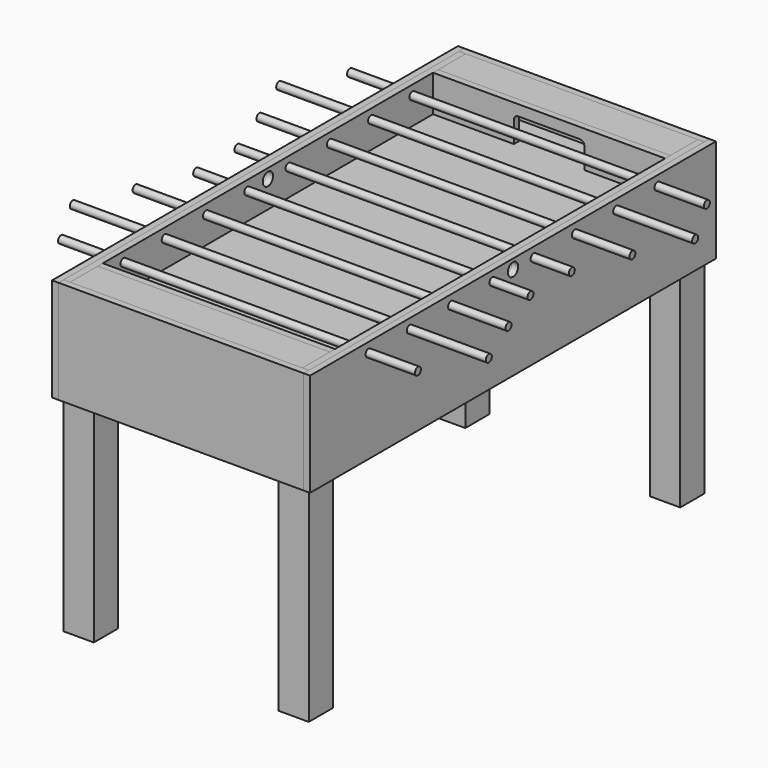
from build123d import *

# Parameters (mm, degrees)
F0_W      = 723.9
F0_H      = 1257.3
F1_DEPTH  = 19.05
F3_DEPTH  = 107.95
F4_DEPTH  = 107.95
F2_W      = 685.8
F2_H      = 19.05
F5_DEPTH  = 107.95
F6_DEPTH  = 107.95
F10_DEPTH = 1257.301
F11_DEPTH = 527.05
F8_R      = 11.1125
F12_DEPTH = 614.3625
F13_DEPTH = 550.8625
F14_DEPTH = 493.7125
F15_W     = 723.9
F15_H     = 1257.3
F15_H_2   = 101.6
F16_DEPTH = 19.05
F17_W     = 19.05
F17_H     = 101.6
F18_DEPTH = 107.95
F19_W     = 685.8
F19_H     = 19.05
F20_DEPTH = 88.9
F21_W     = 88.9
F21_H     = 88.9
F22_DEPTH = 787.4
F23_W     = 685.8
F23_H     = 101.6
F24_DEPTH = 19.05
F26_DEPTH = 304.8
F27_DEPTH = 304.8
F28_DEPTH = 420.624


with BuildPart() as f1:
    # F0 (on Top) → F1 (new body)
    with BuildSketch(Plane.XY):
        with Locations((297.7294597745, 583.4037639737)):
            Rectangle(F0_W, F0_H)
    extrude(amount=-F1_DEPTH)

    # F15 (on face) → F16 (join)
    with BuildSketch(Plane.XY):
        with Locations((297.7294597745, 583.4037639737)):
            Rectangle(F15_W, F15_H)
        with Locations((297.7294597745, -96.0462360263)):
            Rectangle(F15_W, F15_H_2)
        with Locations((297.7294597745, 1262.8537639737)):
            Rectangle(F15_W, F15_H_2)
    extrude(amount=-F16_DEPTH)


with BuildPart() as f3:
    # F2 (on face) → F3 (new body)
    with BuildSketch(Plane.XY):
        Polygon((640.6294597745, -26.1962360263), (640.6294597745, -45.2462360263), (659.6794597745, -45.2462360263), (659.6794597745, 1212.0537639737), (640.6294597745, 1212.0537639737), (640.6294597745, 1193.0037639737), align=None)
    extrude(amount=F3_DEPTH)

    # F17 (on face) → F18 (join, through all)
    with BuildSketch(Plane.XY):
        with Locations((650.1544597745, 1262.8537639737)):
            Rectangle(F17_W, F17_H)
        with Locations((650.1544597745, -96.0462360263)):
            Rectangle(F17_W, F17_H)
    extrude(amount=F18_DEPTH)


with BuildPart() as f4:
    # F2 (on face) → F4 (new body)
    with BuildSketch(Plane.XY):
        Polygon((-64.2205402255, 1212.0537639737), (-64.2205402255, -45.2462360263), (-45.1705402255, -45.2462360263), (-45.1705402255, -26.1962360263), (-45.1705402255, 1193.0037639737), (-45.1705402255, 1212.0537639737), align=None)
    extrude(amount=F4_DEPTH)

    # F17 (on face) → F18, piece 2 (join, through all)
    with BuildSketch(Plane.XY):
        with Locations((-54.6955402255, 1262.8537639737)):
            Rectangle(F17_W, F17_H)
        with Locations((-54.6955402255, -96.0462360263)):
            Rectangle(F17_W, F17_H)
    extrude(amount=F18_DEPTH)


with BuildPart() as f5:
    # F2 (on face) → F5 (new body)
    with BuildSketch(Plane.XY):
        with Locations((297.7294597745, -35.7212360263)):
            Rectangle(F2_W, F2_H)
    extrude(amount=F5_DEPTH)


with BuildPart() as f6:
    # F2 (on face) → F6 (new body)
    with BuildSketch(Plane.XY):
        with Locations((297.7294597745, 1202.5287639737)):
            Rectangle(F2_W, F2_H)
    extrude(amount=F6_DEPTH)


with BuildPart() as f10_tool:
    # F9 (on face) → F10 (new body, through all)
    with BuildSketch(Plane(origin=(0, 1212.0537639737, 0), x_dir=(-1, 0, 0), z_dir=(0, 1, 0))):
        with BuildLine():
            Line((-401.7107097745, 0), (-297.7294597745, 0))
            Line((-297.7294597745, 0), (-297.7294597745, 76.2))
            Line((-297.7294597745, 76.2), (-389.0107097745, 76.2))
            ThreePointArc((-389.0107097745, 76.2), (-397.9909658956, 72.4802561211), (-401.7107097745, 63.5))
            Line((-401.7107097745, 63.5), (-401.7107097745, 0))
        make_face()
        with BuildLine():
            Line((-297.7294597745, 76.2), (-297.7294597745, 0))
            Line((-297.7294597745, 0), (-193.7482097745, 0))
            Line((-193.7482097745, 0), (-193.7482097745, 63.5))
            ThreePointArc((-193.7482097745, 63.5), (-197.4679536534, 72.4802561211), (-206.4482097745, 76.2))
            Line((-206.4482097745, 76.2), (-297.7294597745, 76.2))
        make_face()
    extrude(amount=-F10_DEPTH)


with BuildPart() as f5_1:
    add(f5.part)

    # F10: cut by f10_tool
    add(f10_tool.part, mode=Mode.SUBTRACT)


with BuildPart() as f6_1:
    add(f6.part)

    # F10: cut by f10_tool
    add(f10_tool.part, mode=Mode.SUBTRACT)


with BuildPart() as f11:
    # F8 (on offset) → F11 (new body, symmetric)
    with BuildSketch(Plane.YZ.offset(297.7294597745)):
        with BuildLine():
            ThreePointArc((1127.9162639737, 79.375), (1116.8037639737, 90.4875), (1105.6912639737, 79.375))
            ThreePointArc((1105.6912639737, 79.375), (1116.8037639737, 68.2625), (1127.9162639737, 79.375))
        make_face()
    extrude(amount=F11_DEPTH, both=True)


with BuildPart() as f11b:
    # F8 (on offset) → F11, piece 2 (new body, symmetric)
    with BuildSketch(Plane.YZ.offset(297.7294597745)):
        with Locations((50.0037639737, 79.375)):
            Circle(F8_R)
    extrude(amount=F11_DEPTH, both=True)


with BuildPart() as f12:
    # F8 (on offset) → F12 (new body, symmetric)
    with BuildSketch(Plane.YZ.offset(297.7294597745)):
        with BuildLine():
            Line((964.4037639737, 79.375), (953.2912639737, 79.375))
            ThreePointArc((953.2912639737, 79.375), (964.4037639737, 68.2625), (975.5162639737, 79.375))
            Line((975.5162639737, 79.375), (964.4037639737, 79.375))
        make_face()
        with BuildLine():
            ThreePointArc((975.5162639737, 79.375), (964.4037639737, 90.4875), (953.2912639737, 79.375))
            Line((953.2912639737, 79.375), (964.4037639737, 79.375))
            Line((964.4037639737, 79.375), (975.5162639737, 79.375))
        make_face()
    extrude(amount=F12_DEPTH, both=True)


with BuildPart() as f12b:
    # F8 (on offset) → F12, piece 2 (new body, symmetric)
    with BuildSketch(Plane.YZ.offset(297.7294597745)):
        with BuildLine():
            ThreePointArc((191.2912639737, 79.375), (202.4037639737, 68.2625), (213.5162639737, 79.375))
            Line((213.5162639737, 79.375), (202.4037639737, 79.375))
            Line((202.4037639737, 79.375), (191.2912639737, 79.375))
        make_face()
        with BuildLine():
            Line((202.4037639737, 79.375), (213.5162639737, 79.375))
            ThreePointArc((213.5162639737, 79.375), (202.4037639737, 90.4875), (191.2912639737, 79.375))
            Line((191.2912639737, 79.375), (202.4037639737, 79.375))
        make_face()
    extrude(amount=F12_DEPTH, both=True)


with BuildPart() as f13:
    # F8 (on offset) → F13 (new body, symmetric)
    with BuildSketch(Plane.YZ.offset(297.7294597745)):
        with BuildLine():
            Line((812.0037639737, 79.375), (800.8912639737, 79.375))
            ThreePointArc((800.8912639737, 79.375), (812.0037639737, 68.2625), (823.1162639737, 79.375))
            Line((823.1162639737, 79.375), (812.0037639737, 79.375))
        make_face()
        with BuildLine():
            ThreePointArc((823.1162639737, 79.375), (812.0037639737, 90.4875), (800.8912639737, 79.375))
            Line((800.8912639737, 79.375), (812.0037639737, 79.375))
            Line((812.0037639737, 79.375), (823.1162639737, 79.375))
        make_face()
    extrude(amount=F13_DEPTH, both=True)


with BuildPart() as f13b:
    # F8 (on offset) → F13, piece 2 (new body, symmetric)
    with BuildSketch(Plane.YZ.offset(297.7294597745)):
        with BuildLine():
            Line((354.8037639737, 79.375), (365.9162639737, 79.375))
            ThreePointArc((365.9162639737, 79.375), (354.8037639737, 90.4875), (343.6912639737, 79.375))
            Line((343.6912639737, 79.375), (354.8037639737, 79.375))
        make_face()
        with BuildLine():
            ThreePointArc((343.6912639737, 79.375), (354.8037639737, 68.2625), (365.9162639737, 79.375))
            Line((365.9162639737, 79.375), (354.8037639737, 79.375))
            Line((354.8037639737, 79.375), (343.6912639737, 79.375))
        make_face()
    extrude(amount=F13_DEPTH, both=True)


with BuildPart() as f14:
    # F8 (on offset) → F14 (new body, symmetric)
    with BuildSketch(Plane.YZ.offset(297.7294597745)):
        with BuildLine():
            ThreePointArc((496.0912639737, 79.375), (507.2037639737, 68.2625), (518.3162639737, 79.375))
            Line((518.3162639737, 79.375), (507.2037639737, 79.375))
            Line((507.2037639737, 79.375), (496.0912639737, 79.375))
        make_face()
        with BuildLine():
            Line((507.2037639737, 79.375), (518.3162639737, 79.375))
            ThreePointArc((518.3162639737, 79.375), (507.2037639737, 90.4875), (496.0912639737, 79.375))
            Line((496.0912639737, 79.375), (507.2037639737, 79.375))
        make_face()
    extrude(amount=F14_DEPTH, both=True)


with BuildPart() as f14b:
    # F8 (on offset) → F14, piece 2 (new body, symmetric)
    with BuildSketch(Plane.YZ.offset(297.7294597745)):
        with BuildLine():
            Line((659.6037639737, 79.375), (648.4912639737, 79.375))
            ThreePointArc((648.4912639737, 79.375), (659.6037639737, 68.2625), (670.7162639737, 79.375))
            Line((670.7162639737, 79.375), (659.6037639737, 79.375))
        make_face()
        with BuildLine():
            ThreePointArc((670.7162639737, 79.375), (659.6037639737, 90.4875), (648.4912639737, 79.375))
            Line((648.4912639737, 79.375), (659.6037639737, 79.375))
            Line((659.6037639737, 79.375), (670.7162639737, 79.375))
        make_face()
    extrude(amount=F14_DEPTH, both=True)


with BuildPart() as f20:
    # F19 (on face) → F20 (new body)
    with BuildSketch(Plane.XY):
        with Locations((297.7294597745, -137.3212360263)):
            Rectangle(F19_W, F19_H)
    extrude(amount=F20_DEPTH)


with BuildPart() as f20b:
    # F19 (on face) → F20, piece 2 (new body)
    with BuildSketch(Plane.XY):
        with Locations((297.7294597745, 1304.1287639737)):
            Rectangle(F19_W, F19_H)
    extrude(amount=F20_DEPTH)


with BuildPart() as f22:
    # F21 (on face) → F22 (new body)
    with BuildSketch(Plane(origin=(0, 0, -19.05), x_dir=(1, 0, 0), z_dir=(0, 0, -1))):
        with Locations((-19.7705402255, -1269.2037639737)):
            Rectangle(F21_W, F21_H)
    extrude(amount=F22_DEPTH)


with BuildPart() as f22b:
    # F21 (on face) → F22, piece 2 (new body)
    with BuildSketch(Plane(origin=(0, 0, -19.05), x_dir=(1, 0, 0), z_dir=(0, 0, -1))):
        with Locations((-19.7705402255, 102.3962360263)):
            Rectangle(F21_W, F21_H)
    extrude(amount=F22_DEPTH)


with BuildPart() as f22c:
    # F21 (on face) → F22, piece 3 (new body)
    with BuildSketch(Plane(origin=(0, 0, -19.05), x_dir=(1, 0, 0), z_dir=(0, 0, -1))):
        with Locations((615.2294597745, -1269.2037639737)):
            Rectangle(F21_W, F21_H)
    extrude(amount=F22_DEPTH)


with BuildPart() as f22d:
    # F21 (on face) → F22, piece 4 (new body)
    with BuildSketch(Plane(origin=(0, 0, -19.05), x_dir=(1, 0, 0), z_dir=(0, 0, -1))):
        with Locations((615.2294597745, 102.3962360263)):
            Rectangle(F21_W, F21_H)
    extrude(amount=F22_DEPTH)


with BuildPart() as f24:
    # F23 (on face) → F24 (new body)
    with BuildSketch(Plane.XY.offset(88.9)):
        with Locations((297.7294597745, -96.0462360263)):
            Rectangle(F23_W, F23_H)
    extrude(amount=F24_DEPTH)


with BuildPart() as f24b:
    # F23 (on face) → F24, piece 2 (new body)
    with BuildSketch(Plane.XY.offset(88.9)):
        with Locations((297.7294597745, 1262.8537639737)):
            Rectangle(F23_W, F23_H)
    extrude(amount=F24_DEPTH)


with BuildPart() as f26:
    # F25 (on face) → F26 (new body)
    with BuildSketch(Plane.XY.offset(107.95)):
        Polygon((659.6794597745, -165.8962360263), (659.6794597745, -146.8462360263), (640.6294597745, -146.8462360263), (-45.1705402255, -146.8462360263), (-64.2205402255, -146.8462360263), (-64.2205402255, -165.8962360263), align=None)
    extrude(amount=-F26_DEPTH)


with BuildPart() as f26b:
    # F25 (on face) → F26, piece 2 (new body)
    with BuildSketch(Plane.XY.offset(107.95)):
        Polygon((640.6294597745, 1313.6537639737), (659.6794597745, 1313.6537639737), (659.6794597745, 1332.7037639737), (-64.2205402255, 1332.7037639737), (-64.2205402255, 1313.6537639737), (-45.1705402255, 1313.6537639737), align=None)
    extrude(amount=-F26_DEPTH)


with BuildPart() as f27:
    # F25 (on face) → F27 (new body)
    with BuildSketch(Plane.XY.offset(107.95)):
        Polygon((659.6794597745, 1313.6537639737), (659.6794597745, -146.8462360263), (659.6794597745, -165.8962360263), (678.7294597745, -165.8962360263), (678.7294597745, 1332.7037639737), (659.6794597745, 1332.7037639737), align=None)
    extrude(amount=-F27_DEPTH)


with BuildPart() as f27b:
    # F25 (on face) → F27, piece 2 (new body)
    with BuildSketch(Plane.XY.offset(107.95)):
        Polygon((-83.2705402255, -165.8962360263), (-64.2205402255, -165.8962360263), (-64.2205402255, -146.8462360263), (-64.2205402255, 1313.6537639737), (-64.2205402255, 1332.7037639737), (-83.2705402255, 1332.7037639737), align=None)
    extrude(amount=-F27_DEPTH)


with BuildPart() as f28_tool:
    # F8 (on offset) → F28 (new body, symmetric)
    with BuildSketch(Plane.YZ.offset(297.7294597745)):
        with BuildLine():
            ThreePointArc((564.3537639737, 79.375), (569.9333797921, 65.9046158184), (583.4037639737, 60.325))
            Line((583.4037639737, 60.325), (583.4037639737, 79.375))
            Line((583.4037639737, 79.375), (564.3537639737, 79.375))
        make_face()
        with Locations((50.0037639737, 79.375)):
            Circle(F8_R)
        with BuildLine():
            ThreePointArc((191.2912639737, 79.375), (202.4037639737, 68.2625), (213.5162639737, 79.375))
            Line((213.5162639737, 79.375), (202.4037639737, 79.375))
            Line((202.4037639737, 79.375), (191.2912639737, 79.375))
        make_face()
        with BuildLine():
            Line((202.4037639737, 79.375), (213.5162639737, 79.375))
            ThreePointArc((213.5162639737, 79.375), (202.4037639737, 90.4875), (191.2912639737, 79.375))
            Line((191.2912639737, 79.375), (202.4037639737, 79.375))
        make_face()
        with BuildLine():
            ThreePointArc((343.6912639737, 79.375), (354.8037639737, 68.2625), (365.9162639737, 79.375))
            Line((365.9162639737, 79.375), (354.8037639737, 79.375))
            Line((354.8037639737, 79.375), (343.6912639737, 79.375))
        make_face()
        with BuildLine():
            Line((354.8037639737, 79.375), (365.9162639737, 79.375))
            ThreePointArc((365.9162639737, 79.375), (354.8037639737, 90.4875), (343.6912639737, 79.375))
            Line((343.6912639737, 79.375), (354.8037639737, 79.375))
        make_face()
        with BuildLine():
            ThreePointArc((496.0912639737, 79.375), (507.2037639737, 68.2625), (518.3162639737, 79.375))
            Line((518.3162639737, 79.375), (507.2037639737, 79.375))
            Line((507.2037639737, 79.375), (496.0912639737, 79.375))
        make_face()
        with BuildLine():
            Line((507.2037639737, 79.375), (518.3162639737, 79.375))
            ThreePointArc((518.3162639737, 79.375), (507.2037639737, 90.4875), (496.0912639737, 79.375))
            Line((496.0912639737, 79.375), (507.2037639737, 79.375))
        make_face()
        with BuildLine():
            ThreePointArc((1127.9162639737, 79.375), (1116.8037639737, 90.4875), (1105.6912639737, 79.375))
            ThreePointArc((1105.6912639737, 79.375), (1116.8037639737, 68.2625), (1127.9162639737, 79.375))
        make_face()
        with BuildLine():
            ThreePointArc((975.5162639737, 79.375), (964.4037639737, 90.4875), (953.2912639737, 79.375))
            Line((953.2912639737, 79.375), (964.4037639737, 79.375))
            Line((964.4037639737, 79.375), (975.5162639737, 79.375))
        make_face()
        with BuildLine():
            Line((964.4037639737, 79.375), (953.2912639737, 79.375))
            ThreePointArc((953.2912639737, 79.375), (964.4037639737, 68.2625), (975.5162639737, 79.375))
            Line((975.5162639737, 79.375), (964.4037639737, 79.375))
        make_face()
        with BuildLine():
            ThreePointArc((823.1162639737, 79.375), (812.0037639737, 90.4875), (800.8912639737, 79.375))
            Line((800.8912639737, 79.375), (812.0037639737, 79.375))
            Line((812.0037639737, 79.375), (823.1162639737, 79.375))
        make_face()
        with BuildLine():
            Line((812.0037639737, 79.375), (800.8912639737, 79.375))
            ThreePointArc((800.8912639737, 79.375), (812.0037639737, 68.2625), (823.1162639737, 79.375))
            Line((823.1162639737, 79.375), (812.0037639737, 79.375))
        make_face()
        with BuildLine():
            ThreePointArc((670.7162639737, 79.375), (659.6037639737, 90.4875), (648.4912639737, 79.375))
            Line((648.4912639737, 79.375), (659.6037639737, 79.375))
            Line((659.6037639737, 79.375), (670.7162639737, 79.375))
        make_face()
        with BuildLine():
            Line((659.6037639737, 79.375), (648.4912639737, 79.375))
            ThreePointArc((648.4912639737, 79.375), (659.6037639737, 68.2625), (670.7162639737, 79.375))
            Line((670.7162639737, 79.375), (659.6037639737, 79.375))
        make_face()
        with BuildLine():
            Line((583.4037639737, 79.375), (583.4037639737, 60.325))
            ThreePointArc((583.4037639737, 60.325), (596.8741481553, 65.9046158184), (602.4537639737, 79.375))
            Line((602.4537639737, 79.375), (583.4037639737, 79.375))
        make_face()
        with BuildLine():
            Line((564.3537639737, 79.375), (583.4037639737, 79.375))
            Line((583.4037639737, 79.375), (602.4537639737, 79.375))
            ThreePointArc((602.4537639737, 79.375), (583.4037639737, 98.425), (564.3537639737, 79.375))
        make_face()
    extrude(amount=F28_DEPTH, both=True)


with BuildPart() as f3_1:
    add(f3.part)

    # F28: cut by f28_tool
    add(f28_tool.part, mode=Mode.SUBTRACT)


with BuildPart() as f4_1:
    add(f4.part)

    # F28: cut by f28_tool
    add(f28_tool.part, mode=Mode.SUBTRACT)


with BuildPart() as f27_1:
    add(f27.part)

    # F28: cut by f28_tool
    add(f28_tool.part, mode=Mode.SUBTRACT)


with BuildPart() as f27b_1:
    add(f27b.part)

    # F28: cut by f28_tool
    add(f28_tool.part, mode=Mode.SUBTRACT)


solid = Compound([f1.part, f5_1.part, f6_1.part, f11.part, f11b.part, f12.part, f12b.part, f13.part, f13b.part, f14.part, f14b.part, f20.part, f20b.part, f22.part, f22b.part, f22c.part, f22d.part, f24.part, f24b.part, f26.part, f26b.part, f3_1.part, f4_1.part, f27_1.part, f27b_1.part])
